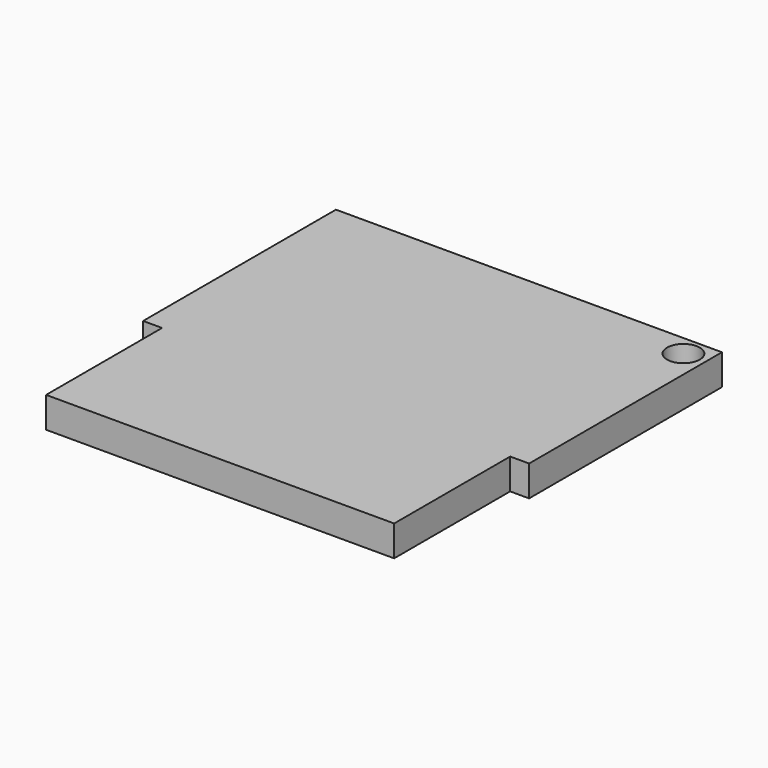
from build123d import *

# Parameters (mm, degrees)
F1_DEPTH     = 11.938
F2_R         = 6.35
F3_DEPTH     = 25.4
F4_TEXT_SIZE = 29.2936184754
F5_DEPTH     = 15
F7_DEPTH     = 3.048
F8_W         = 63.5
F8_H         = 19.6682121078
F9_DEPTH     = 5.08
F10_W        = 30.6565033495
F10_H        = 19.6682121078
F11_DEPTH    = 9.144


# Not quite as in the source:
# - Text() gives the source's letters only with a copy of the font that has no kerning and outlines rounded to 1/6400 em; it was checked with that copy


with BuildPart() as f1:
    # F0 (on Top) → F1 (new body)
    with BuildSketch(Plane.XY):
        Polygon((-67.634, -75), (67.634, -75), (67.634, -18.659574911), (75, -18.659574911), (75, 75), (-75, 75), (-75, -18.659574911), (-67.634, -18.659574911), align=None)
    extrude(amount=F1_DEPTH)

    # F2 (on face) → F3 (cut)
    with BuildSketch(Plane.XY.offset(11.938)):
        with Locations((66.4393976331, 67.0048370957)):
            Circle(F2_R)
    extrude(amount=-F3_DEPTH, mode=Mode.SUBTRACT)

    # F4 (on face) → F5 (join)
    with BuildSketch(Plane.XY.offset(11.938)):
        with Locations((-52.7188277338, 43.6495803297)):
            Text('HCTIWS', F4_TEXT_SIZE, font='Open Sans', font_style=FontStyle.BOLDITALIC, text_align=(TextAlign.LEFT, TextAlign.BOTTOM))
    extrude(amount=-F5_DEPTH)

    # F6 (on face) → F7 (join)
    with BuildSketch(Plane(origin=(0, 0, 0), x_dir=(1, 0, 0), z_dir=(0, 0, -1))):
        Polygon((-5.0510223955, -34.8242968321), (0, -34.8242968321), (0, 0), (7.8365136163, 0), (-2.7162800543, 18.2779747993), (-13.2690737249, 0), (-5.0510223955, 0), align=None)
    extrude(amount=F7_DEPTH)

    # F8 (on face) → F9 (cut)
    with BuildSketch(Plane(origin=(0, 0, 0), x_dir=(1, 0, 0), z_dir=(0, 0, -1))):
        with Locations((-1.0934966505, 33.664283369)):
            Rectangle(F8_W, F8_H)
    extrude(amount=-F9_DEPTH, mode=Mode.SUBTRACT)

    # F10 (on face) → F11 (join)
    with BuildSketch(Plane(origin=(0, 0, 5.08), x_dir=(1, 0, 0), z_dir=(0, 0, -1))):
        with Locations((15.3282516748, 33.664283369)):
            Rectangle(F10_W, F10_H)
    extrude(amount=F11_DEPTH)


solid = f1.part
